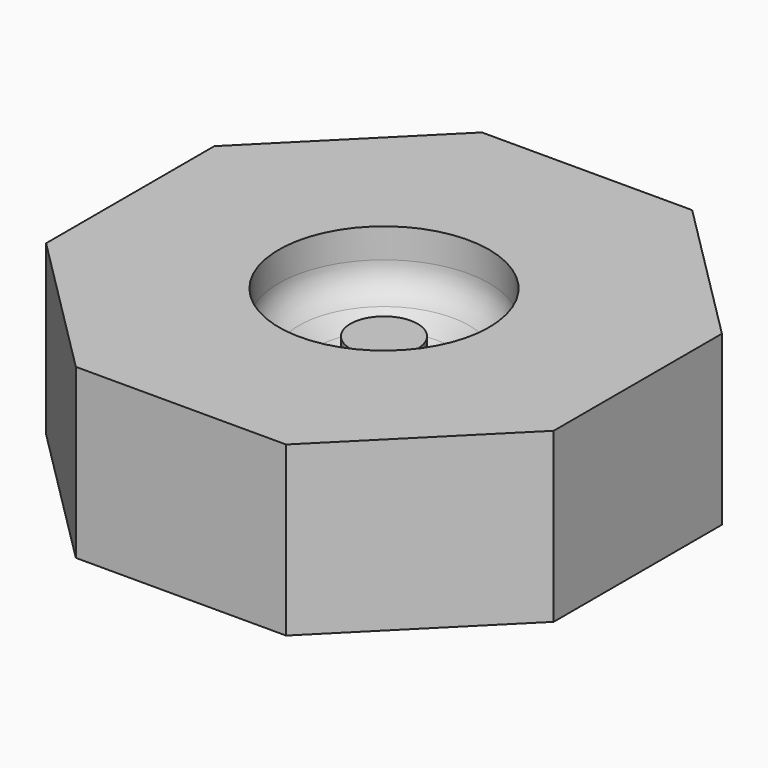
from build123d import *

# Parameters (mm, degrees)
F1_DEPTH  = 50.8
F2_R      = 31.75
F3_DEPTH  = 19.05
F4_R      = 12.7
F5_DEPTH  = 38.1
F6_R      = 22.225
F7_DEPTH  = 25.4
F11_R     = 10.16
F12_DEPTH = 25.4


# Not quite as in the source:
# - a fillet or chamfer that OpenCascade refuses, or shapes differently, is made with other operations: its cross-section is extruded or revolved along the edge and cut away or added


with BuildPart() as f1:
    # F0 (on Top) → F1 (new body)
    with BuildSketch(Plane.XY):
        Polygon((76.6512806053, -31.75), (76.6512806053, 31.75), (31.75, 76.6512806053), (-31.75, 76.6512806053), (-76.6512806053, 31.75), (-76.6512806053, -31.75), (-31.75, -76.6512806053), (31.75, -76.6512806053), align=None)
    extrude(amount=F1_DEPTH)

    # F2 (on face) → F3 (cut)
    with BuildSketch(Plane.XY.offset(50.8)):
        Circle(F2_R)
    extrude(amount=-F3_DEPTH, mode=Mode.SUBTRACT)

    # F4 (on face) → F5 (cut)
    with BuildSketch(Plane.XY.offset(50.8)):
        Circle(F4_R)
    extrude(amount=-F5_DEPTH, mode=Mode.SUBTRACT)

    # F6 (on face) → F7 (cut)
    with BuildSketch(Plane.XY.offset(50.8)):
        Circle(F6_R)
    extrude(amount=-F7_DEPTH, mode=Mode.SUBTRACT)

    # F8: fillet of radius 10.16 on 1 edges, made by hand

    # F8_s1 → F8_t2 (revolve)
    with BuildSketch(Plane.XZ):
        with BuildLine():
            ThreePointArc((31.75, 41.8901368334), (28.9953089065, 34.9340603531), (22.225, 31.75))
            Line((22.225, 31.75), (31.75, 31.75))
            Line((31.75, 31.75), (31.75, 41.8901368334))
        make_face()
    revolve(axis=Axis((0, 0, 31.75), (0, 0, 1)))

    # F9: fillet of radius 10.16 on 1 edges, made by hand

    # F9_s1 → F9_t2 (revolve)
    with BuildSketch(Plane.XZ):
        with BuildLine():
            ThreePointArc((22.225, 31.75), (18.4860405842, 27.1357730325), (12.8064279214, 25.4))
            Line((12.8064279214, 25.4), (22.225, 25.4))
            Line((22.225, 25.4), (22.225, 31.75))
        make_face()
    revolve(axis=Axis((0, 0, 25.4), (0, 0, 1)))

    # F10: chamfer of 10.16 on 1 edges, made by hand

    # F10_s1 → F10_t2 (revolve, cut)
    with BuildSketch(Plane.XZ):
        with BuildLine():
            Line((26.0358422648, 32.838882269), (19.9865565056, 28.4792884435))
            Line((19.9865565056, 28.4792884435), (19.8363599068, 28.6161504971))
            ThreePointArc((19.8363599068, 28.6161504971), (21.1312925718, 30.0979038097), (22.0366285584, 31.8262))
            Line((22.0366285584, 31.8262), (22.2123, 31.9528027367))
            ThreePointArc((22.2123, 31.9528027367), (24.1382310347, 32.2649415193), (25.9535194466, 33.0246595378))
            Line((25.9535194466, 33.0246595378), (26.0358422648, 32.838882269))
        make_face()
    revolve(axis=Axis((0, 0, 31.75), (0, 0, 1)), mode=Mode.SUBTRACT)

    # F11 (on face) → F12 (join)
    with BuildSketch(Plane.XY.offset(12.7)):
        Circle(F11_R)
    extrude(amount=F12_DEPTH)


solid = f1.part
